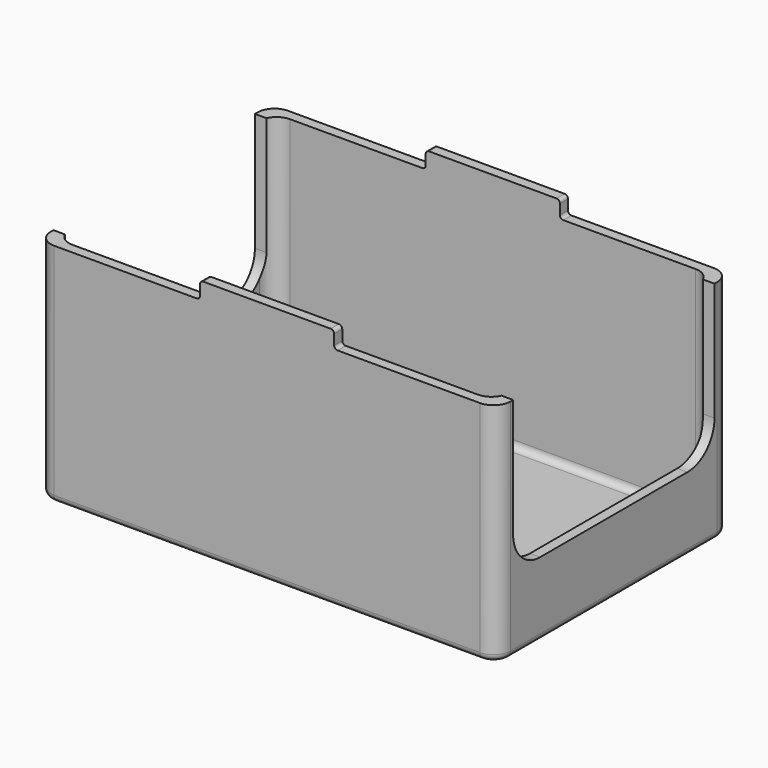
from build123d import *

# Parameters (mm, degrees)
F0_R     = 3
F0_R_2   = 1.4
F0_R_3   = 17.5
F0_R_4   = 1.5
F1_DEPTH = 3
F0_W     = 65
F0_H     = 3
F2_DEPTH = 67
F4_DEPTH = 136.001
F5_W     = 39.7
F5_H     = 3
F6_W     = 39.7
F6_H     = 3
F7_DEPTH = 5
F8_R     = 1
F9_R     = 5
F10_R    = 2


# Not quite as in the source:
# - a feature names something its author has since deleted; it is built from what else it names


with BuildPart() as f1:
    # F0 (on Top) → F1 (new body)
    with BuildSketch(Plane.XY):
        Polygon((-60.3749420391, 27.6098903269), (-60.3749420391, 7), (-15.3749420391, 7), (-15.3749420391, 12), (24.6250579609, 12), (24.6250579609, 7), (69.6250579609, 7), (69.6250579609, 53.4099719524), (69.6250579609, 87.5), (4.6250579609, 87.5), (-60.3749420391, 87.5), (-60.3749420391, 71.25), align=None)
        with Locations((-30.3749420391, 23.25)):
            Circle(F0_R, mode=Mode.SUBTRACT)
        with Locations((-11.3749420391, 31.25)):
            Circle(F0_R_2, mode=Mode.SUBTRACT)
        with Locations((20.6250579609, 31.25)):
            Circle(F0_R_2, mode=Mode.SUBTRACT)
        with Locations((52.6250579609, 23.25)):
            Circle(F0_R, mode=Mode.SUBTRACT)
        with Locations((-11.3749420391, 63.25)):
            Circle(F0_R_2, mode=Mode.SUBTRACT)
        with BuildLine():
            ThreePointArc((-27.3749420391, 71.25), (-30.3749420391, 68.25), (-33.3749420391, 71.25))
            ThreePointArc((-33.3749420391, 71.25), (-30.3749420391, 74.25), (-27.3749420391, 71.25))
        make_face(mode=Mode.SUBTRACT)
        with Locations((4.6250579609, 47.25)):
            Circle(F0_R_3, mode=Mode.SUBTRACT)
        with Locations((20.6250579609, 63.25)):
            Circle(F0_R_2, mode=Mode.SUBTRACT)
        with Locations((52.6250579609, 71.25)):
            Circle(F0_R, mode=Mode.SUBTRACT)
        Polygon((-15.3749420391, 12), (-15.3749420391, 7), (14.8769766092, 7), (24.6250579609, 7), (24.6250579609, 12), align=None)
        with BuildLine():
            ThreePointArc((-27.3749420391, 71.25), (-30.3749420391, 74.25), (-33.3749420391, 71.25))
            ThreePointArc((-33.3749420391, 71.25), (-30.3749420391, 68.25), (-27.3749420391, 71.25))
        make_face()
        with BuildLine():
            ThreePointArc((-28.8749420391, 71.25), (-30.3749420391, 69.75), (-31.8749420391, 71.25))
            ThreePointArc((-31.8749420391, 71.25), (-30.3749420391, 72.75), (-28.8749420391, 71.25))
        make_face(mode=Mode.SUBTRACT)
        with BuildLine():
            ThreePointArc((-28.8749420391, 71.25), (-30.3749420391, 72.75), (-31.8749420391, 71.25))
            ThreePointArc((-31.8749420391, 71.25), (-30.3749420391, 69.75), (-28.8749420391, 71.25))
        make_face()
        with Locations((52.6250579609, 71.25)):
            Circle(F0_R)
        with Locations((52.6250579609, 71.25)):
            Circle(F0_R_4, mode=Mode.SUBTRACT)
        with Locations((52.6250579609, 71.25)):
            Circle(F0_R_4)
        with Locations((52.6250579609, 23.25)):
            Circle(F0_R)
        with Locations((52.6250579609, 23.25)):
            Circle(F0_R_4, mode=Mode.SUBTRACT)
        with Locations((52.6250579609, 23.25)):
            Circle(F0_R_4)
        with Locations((-30.3749420391, 23.25)):
            Circle(F0_R)
        with Locations((-30.3749420391, 23.25)):
            Circle(F0_R_4, mode=Mode.SUBTRACT)
        with Locations((-30.3749420391, 23.25)):
            Circle(F0_R_4)
    extrude(amount=F1_DEPTH)

    # F0 (on Top) → F2 (join)
    with BuildSketch(Plane.XY):
        Polygon((-63.3749420391, 27.6098903269), (-60.3749420391, 27.6098903269), (-60.3749420391, 71.25), (-60.3749420391, 87.5), (-60.3749420391, 90.5), (-63.3749420391, 90.5), align=None)
        with Locations((-27.8749420391, 89)):
            Rectangle(F0_W, F0_H)
        with Locations((37.1250579609, 89)):
            Rectangle(F0_W, F0_H)
        Polygon((69.6250579609, 87.5), (69.6250579609, 53.4099719524), (72.6250579609, 53.4099719524), (72.6250579609, 90.5), (69.6250579609, 90.5), align=None)
        Polygon((69.6250579609, 7), (69.6250579609, 4), (72.6250579609, 4), (72.6250579609, 53.4099719524), (69.6250579609, 53.4099719524), align=None)
        Polygon((14.8769766092, 4), (69.6250579609, 4), (69.6250579609, 7), (24.6250579609, 7), (14.8769766092, 7), align=None)
        Polygon((-60.3749420391, 7), (-60.3749420391, 4), (14.8769766092, 4), (14.8769766092, 7), (-15.3749420391, 7), align=None)
        Polygon((-63.3749420391, 4), (-60.3749420391, 4), (-60.3749420391, 7), (-60.3749420391, 27.6098903269), (-63.3749420391, 27.6098903269), align=None)
    extrude(amount=F2_DEPTH)

    # F3 (on face) → F4 (cut, through all)
    with BuildSketch(Plane(origin=(-63.3749420391, 0, 0), x_dir=(0, -1, 0), z_dir=(-1, 0, 0))):
        with BuildLine():
            ThreePointArc((-20, 21.9706685841), (-12.9289321881, 24.8996007722), (-10, 31.9706685841))
            ThreePointArc((-10, 31.9706685841), (-20, 41.9706685841), (-30, 31.9706685841))
            ThreePointArc((-30, 31.9706685841), (-27.0710678119, 24.8996007722), (-20, 21.9706685841))
        make_face()
        with BuildLine():
            ThreePointArc((-30, 31.9706685841), (-20, 41.9706685841), (-10, 31.9706685841))
            Line((-10, 31.9706685841), (-10, 67))
            Line((-10, 67), (-30, 67))
            Line((-30, 67), (-30, 31.9706685841))
        make_face()
        with BuildLine():
            ThreePointArc((-74.5, 21.9706685841), (-67.4289321881, 24.8996007722), (-64.5, 31.9706685841))
            ThreePointArc((-64.5, 31.9706685841), (-74.5, 41.9706685841), (-84.5, 31.9706685841))
            ThreePointArc((-84.5, 31.9706685841), (-81.5710678119, 24.8996007722), (-74.5, 21.9706685841))
        make_face()
        with BuildLine():
            Line((-64.5, 31.9706685841), (-30, 31.9706685841))
            Line((-30, 31.9706685841), (-30, 67))
            Line((-30, 67), (-84.5, 67))
            Line((-84.5, 67), (-84.5, 31.9706685841))
            ThreePointArc((-84.5, 31.9706685841), (-74.5, 41.9706685841), (-64.5, 31.9706685841))
        make_face()
        with BuildLine():
            ThreePointArc((-20, 21.9706685841), (-27.0710678119, 24.8996007722), (-30, 31.9706685841))
            Line((-30, 31.9706685841), (-64.5, 31.9706685841))
            ThreePointArc((-64.5, 31.9706685841), (-67.4289321881, 24.8996007722), (-74.5, 21.9706685841))
            Line((-74.5, 21.9706685841), (-20, 21.9706685841))
        make_face()
    extrude(amount=-F4_DEPTH, mode=Mode.SUBTRACT)

    # F5 (on face) + F6 (on face) → F7 (join)
    with BuildSketch(Plane.XY.offset(67)):
        with Locations((4.6250579609, 5.5)):
            Rectangle(F5_W, F5_H)
    with BuildSketch(Plane.XY.offset(67)):
        with Locations((4.6250579609, 89)):
            Rectangle(F6_W, F6_H)
    extrude(amount=F7_DEPTH)

    # F8
    f8_edges = [f1.edges().sort_by_distance(p)[0] for p in [
        (-15.224942, 5.5, 67),
        (-15.224942, 5.5, 72),
        (24.475058, 5.5, 72),
        (24.475058, 5.5, 67),
        (-15.224942, 89, 67),
        (-15.224942, 89, 72),
        (24.475058, 89, 72),
        (24.475058, 89, 67),
    ]]
    fillet(f8_edges, radius=F8_R)

    # F9
    f9_edges = [f1.edges().sort_by_distance(p)[0] for p in [
        (72.625058, 4, 33.5),
        (72.625058, 90.5, 33.5),
        (-63.374942, 90.5, 33.5),
        (-63.374942, 4, 33.5),
        (-60.374942, 7, 35),
        (-60.374942, 87.5, 35),
        (69.625058, 87.5, 35),
        (69.625058, 7, 35),
    ]]
    fillet(f9_edges, radius=F9_R)

    # F10
    f10_edges = [f1.edges().sort_by_distance(p)[0] for p in [
        (4.625058, 87.5, 3),
        (4.625058, 4, 0),
    ]]
    fillet(f10_edges, radius=F10_R)


solid = f1.part
